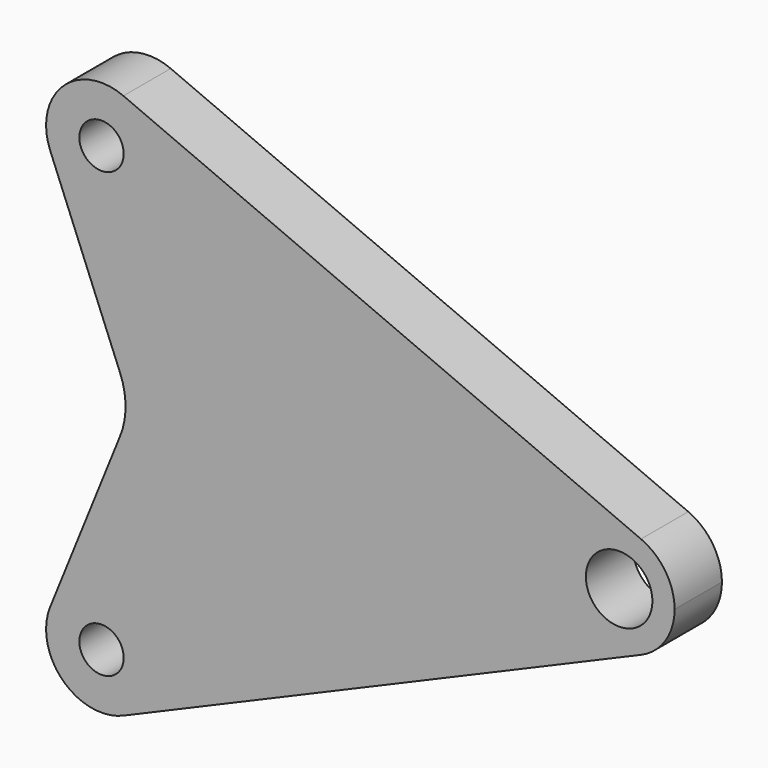
from build123d import *

# Parameters (mm, degrees)
F0_R     = 3
F0_R_2   = 4.5
F1_DEPTH = 8
F2_R     = 10
F4_DEPTH = 4.5
F5_SIZE2 = 4.49999
F5_SIZE  = 1.99999


# Not quite as in the source:
# - a fillet or chamfer is up to 0.001 mm smaller than in the source, because OpenCascade refuses the exact size


with BuildPart() as f1:
    # F0 (on Front) → F1 (new body)
    with BuildSketch(Plane.XZ):
        with BuildLine():
            ThreePointArc((-6.9538789093, 27.1904505494), (1.4310674653, 22.6377961241), (7.5, 30))
            ThreePointArc((7.5, 30), (6.2613081918, 34.1286825656), (2.9543947393, 36.8935877251))
            ThreePointArc((2.9543947393, 36.8935877251), (-5.247540964, 35.3584805524), (-6.9538789093, 27.1904505494))
        make_face()
        with Locations((0, 30)):
            Circle(F0_R, mode=Mode.SUBTRACT)
        with BuildLine():
            ThreePointArc((2.9543947393, 36.8935877251), (6.2613081918, 34.1286825656), (7.5, 30))
            ThreePointArc((7.5, 30), (1.4310674653, 22.6377961241), (-6.9538789093, 27.1904505494))
            Line((-6.9538789093, 27.1904505494), (4.031776205, 0))
            Line((4.031776205, 0), (-6.9538789093, -27.1904505494))
            ThreePointArc((-6.9538789093, -27.1904505494), (1.4310674653, -22.6377961241), (7.5, -30))
            ThreePointArc((7.5, -30), (6.2613081918, -34.1286825656), (2.9543947393, -36.8935877251))
            Line((2.9543947393, -36.8935877251), (72.9543947393, -6.8935877251))
            ThreePointArc((72.9543947393, -6.8935877251), (62.5, 0), (72.9543947393, 6.8935877251))
            Line((72.9543947393, 6.8935877251), (2.9543947393, 36.8935877251))
        make_face()
        with BuildLine():
            ThreePointArc((77.5, 0), (76.2613081918, 4.1286825656), (72.9543947393, 6.8935877251))
            ThreePointArc((72.9543947393, 6.8935877251), (62.5, 0), (72.9543947393, -6.8935877251))
            ThreePointArc((72.9543947393, -6.8935877251), (76.2613081918, -4.1286825656), (77.5, 0))
        make_face()
        with Locations((70, 0)):
            Circle(F0_R_2, mode=Mode.SUBTRACT)
        with BuildLine():
            ThreePointArc((7.5, -30), (1.4310674653, -22.6377961241), (-6.9538789093, -27.1904505494))
            ThreePointArc((-6.9538789093, -27.1904505494), (-5.247540964, -35.3584805524), (2.9543947393, -36.8935877251))
            ThreePointArc((2.9543947393, -36.8935877251), (6.2613081918, -34.1286825656), (7.5, -30))
        make_face()
        with Locations((0, -30)):
            Circle(F0_R, mode=Mode.SUBTRACT)
    extrude(amount=F1_DEPTH)

    # F2
    f2_edges = [f1.edges().sort_by_distance(p)[0] for p in [
        (4.031776, -4, 0),
    ]]
    fillet(f2_edges, radius=F2_R)

    # F3 (on Front) → F4 (cut)
    with BuildSketch(Plane.XZ):
        with BuildLine():
            Line((12.5995942419, 16.7481284808), (17.8527685007, 3.7460659342))
            ThreePointArc((17.8527685007, 3.7460659342), (18.580929955, 0), (17.8527685007, -3.7460659342))
            Line((17.8527685007, -3.7460659342), (12.5995942419, -16.7481284808))
            ThreePointArc((12.5995942419, -16.7481284808), (13.0546176939, -18.926269815), (15.2418005482, -19.3356317277))
            Line((15.2418005482, -19.3356317277), (53.9242593693, -2.7574350901))
            ThreePointArc((53.9242593693, -2.7574350901), (55.7425014736, 0), (53.9242593693, 2.7574350901))
            Line((53.9242593693, 2.7574350901), (15.2418005482, 19.3356317277))
            ThreePointArc((15.2418005482, 19.3356317277), (13.0546176939, 18.926269815), (12.5995942419, 16.7481284808))
        make_face()
    extrude(amount=F4_DEPTH, mode=Mode.SUBTRACT)

    # F5 (size 2 and 4.5 in the source; OpenCascade refuses exactly that, so slightly less here)
    f5_edges = [f1.edges().sort_by_distance(p)[0] for p in [
        (34.58303, -4.5, 11.046533),
    ]]
    f5_side = f1.faces().sort_by_distance((30.018515, -4.5, 0))[0]
    chamfer(f5_edges, length=F5_SIZE, length2=F5_SIZE2, reference=f5_side)


solid = f1.part
